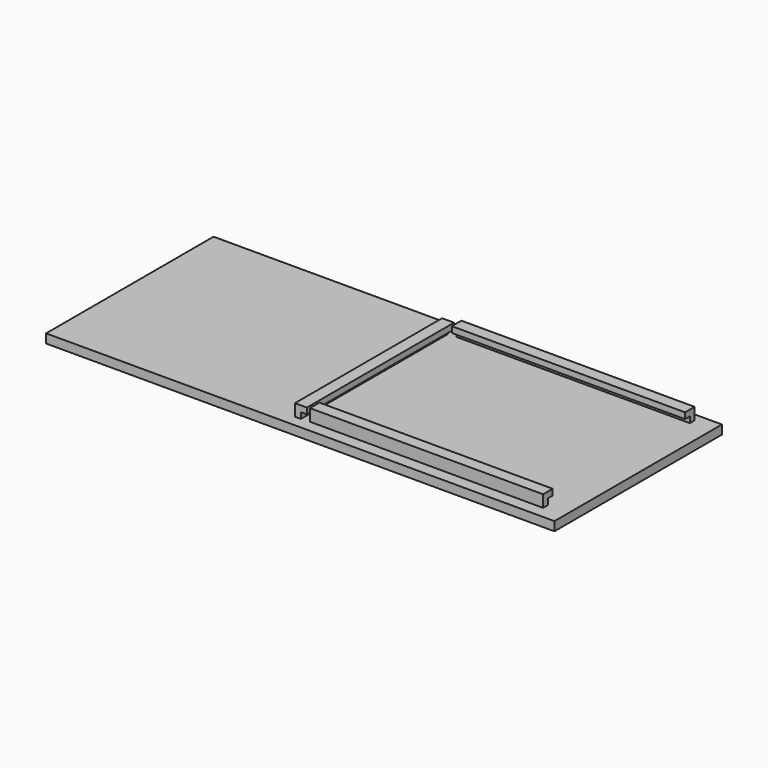
from build123d import *

# Parameters (mm, degrees)
F0_W     = 4
F0_H     = 61.5
F0_W_2   = 78
F0_H_2   = 4
F1_DEPTH = 3
F2_DEPTH = 7
F3_W     = 2
F3_H     = 2
F4_DEPTH = 77.9
F5_W     = 2
F5_H     = 2
F6_DEPTH = 64.1
F7_W     = 2
F7_H     = 2
F8_DEPTH = 78


# Not quite as in the source:
# - a feature names something its author has since deleted; it is built from what else it names


with BuildPart() as f1:
    # F0 (on Top) → F1 (new body)
    with BuildSketch(Plane.XY):
        Polygon((85, 35), (-85, 35), (-85, -25.7047470659), (-85, -35), (-7, -35), (85, -35), align=None)
        with Locations((-2.7990786843, -0.482085079)):
            Rectangle(F0_W, F0_H, mode=Mode.SUBTRACT)
        with Locations((39, -28.9953801334)):
            Rectangle(F0_W_2, F0_H_2, mode=Mode.SUBTRACT)
        with Locations((39, 30.3457357436)):
            Rectangle(F0_W_2, F0_H_2, mode=Mode.SUBTRACT)
    extrude(amount=F1_DEPTH)

    # F0 (on Top) → F2 (join)
    with BuildSketch(Plane.XY):
        with Locations((-2.7990786843, -0.482085079)):
            Rectangle(F0_W, F0_H)
        with Locations((39, -28.9953801334)):
            Rectangle(F0_W_2, F0_H_2)
        with Locations((39, 30.3457357436)):
            Rectangle(F0_W_2, F0_H_2)
    extrude(amount=F2_DEPTH)

    # F3 (on face) → F4 (cut)
    with BuildSketch(Plane.YZ.offset(78)):
        with Locations((-27.9953801334, 4)):
            Rectangle(F3_W, F3_H)
    extrude(amount=-F4_DEPTH, mode=Mode.SUBTRACT)

    # F5 (on face) → F6 (cut)
    with BuildSketch(Plane.XZ.offset(31.232085079)):
        with Locations((-1.7990786843, 4)):
            Rectangle(F5_W, F5_H)
    extrude(amount=-F6_DEPTH, mode=Mode.SUBTRACT)

    # F7 (on face) → F8 (cut)
    with BuildSketch(Plane.YZ.offset(78)):
        with Locations((29.3457357436, 4)):
            Rectangle(F7_W, F7_H)
    extrude(amount=-F8_DEPTH, mode=Mode.SUBTRACT)


solid = f1.part
